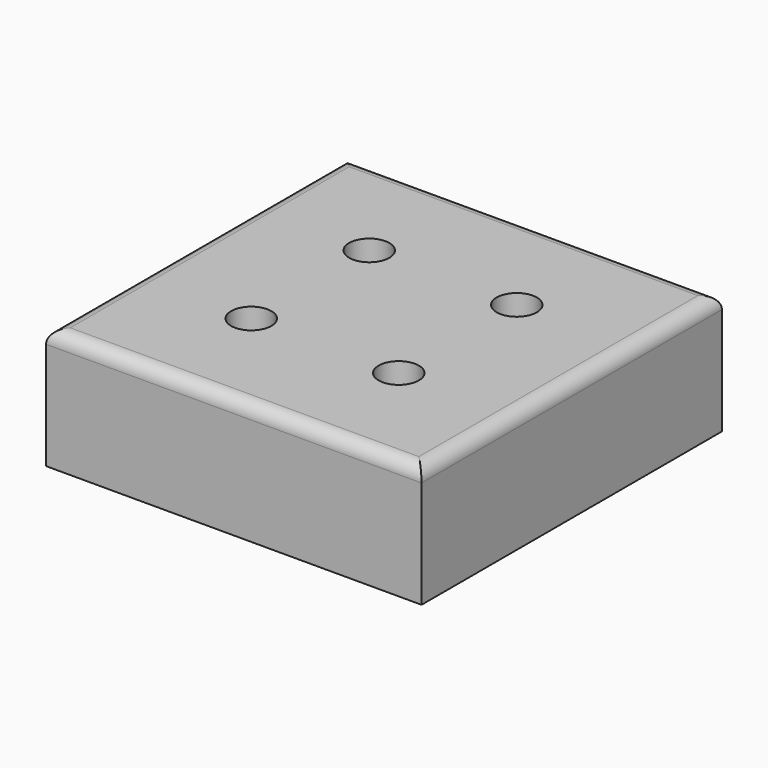
from build123d import *

# Parameters (mm, degrees)
F0_W     = 28
F0_H     = 28
F1_DEPTH = 9
F3_D     = 3
F4_R     = 1


# Not quite as in the source:
# - a feature names something its author has since deleted; it is built from what else it names


with BuildPart() as f1:
    # F0 (on Top) → F1 (new body)
    with BuildSketch(Plane.XY):
        Rectangle(F0_W, F0_H)
    extrude(amount=F1_DEPTH)

    # F3 (through all)
    with Locations(Plane.XY.offset(9)):
        with Locations((5.5, 5.5), (-5.5, 5.5), (-5.5, -5.5), (5.5, -5.5)):
            Hole(F3_D / 2)

    # F4
    f4_edges = [f1.edges().sort_by_distance(p)[0] for p in [
        (0, 14, 9),
        (-14, 0, 9),
        (0, -14, 9),
        (14, 0, 9),
    ]]
    fillet(f4_edges, radius=F4_R)


solid = f1.part
